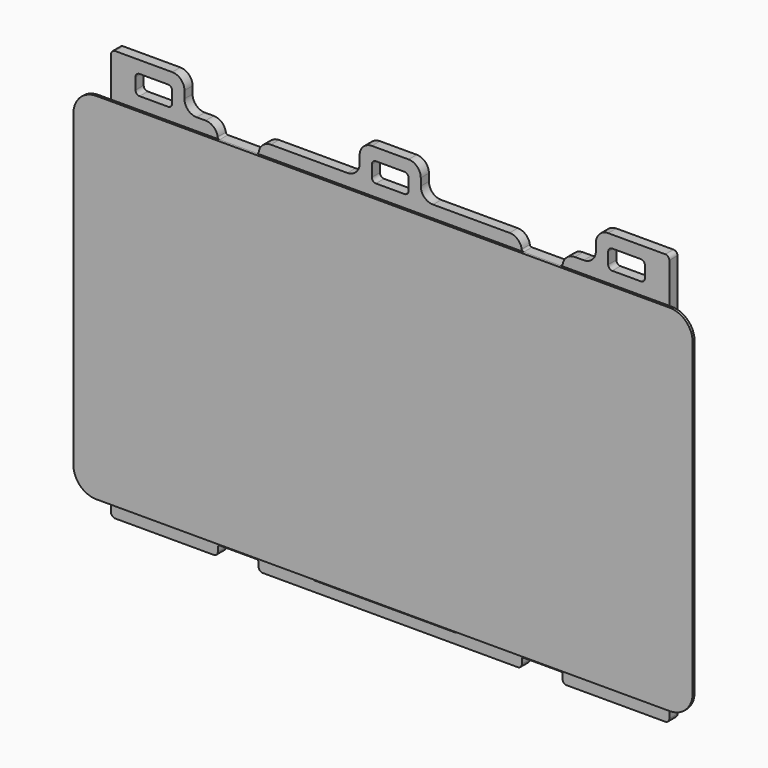
from build123d import *

# Parameters (mm, degrees)
F1_DEPTH   = 0.762
F2_W       = 166.2938
F2_H       = 100.7999
F3_DEPTH   = 5.08
F4_W       = 14.478
F4_H       = 7.874
F4_R       = 1.27
F4_W_2     = 7.874
F4_H_2     = 14.478
F5_DEPTH   = 2.413
F6_SIZE2   = 3.80999
F6_SIZE    = 2.41299
F6_2_SIZE2 = 3.80999
F6_2_SIZE  = 2.41299
F6_3_SIZE2 = 3.80999
F6_3_SIZE  = 2.41299
F6_4_SIZE2 = 3.80999
F6_4_SIZE  = 2.41299
F6_5_SIZE2 = 3.80999
F6_5_SIZE  = 2.41299
F6_6_SIZE2 = 3.80999
F6_6_SIZE  = 2.41299
F6_7_SIZE2 = 3.80999
F6_7_SIZE  = 2.41299
F6_8_SIZE2 = 3.80999
F6_8_SIZE  = 2.41299
F6_9_SIZE2 = 3.80999
F6_9_SIZE  = 2.41299
F7_SIZE2   = 3.80999
F7_SIZE    = 2.41299
F7_2_SIZE2 = 3.80999
F7_2_SIZE  = 2.41299
F7_3_SIZE2 = 3.80999
F7_3_SIZE  = 2.41299
F7_4_SIZE2 = 3.80999
F7_4_SIZE  = 2.41299
F7_5_SIZE2 = 3.80999
F7_5_SIZE  = 2.41299
F7_6_SIZE2 = 3.80999
F7_6_SIZE  = 2.41299
F7_7_SIZE2 = 3.80999
F7_7_SIZE  = 2.41299
F9_DEPTH   = 73.533
F11_DEPTH  = 64.2493
F12_W      = 40.005
F12_H      = 5.08
F13_DEPTH  = 3.2131
F15_DEPTH  = 3.175
F18_DEPTH  = 3.175
F19_R      = 0.635
F19_2_R    = 0.635


# Not quite as in the source:
# - a fillet or chamfer is up to 0.001 mm smaller than in the source, because OpenCascade refuses the exact size


with BuildPart() as f1:
    # F0 (on Front) → F1 (new body)
    with BuildSketch(Plane.XZ):
        with BuildLine():
            ThreePointArc((96.4565, 48.1965), (94.3734434278, 53.2254434278), (89.3445, 55.3085))
            Line((89.3445, 55.3085), (-89.3445, 55.3085))
            ThreePointArc((-89.3445, 55.3085), (-94.3734434278, 53.2254434278), (-96.4565, 48.1965))
            Line((-96.4565, 48.1965), (-96.4565, -48.1965))
            ThreePointArc((-96.4565, -48.1965), (-94.3734434278, -53.2254434278), (-89.3445, -55.3085))
            Line((-89.3445, -55.3085), (89.3445, -55.3085))
            ThreePointArc((89.3445, -55.3085), (94.3734434278, -53.2254434278), (96.4565, -48.1965))
            Line((96.4565, -48.1965), (96.4565, 48.1965))
        make_face()
    extrude(amount=F1_DEPTH)

    # F2 (on face) → F3 (join)
    with BuildSketch(Plane(origin=(0, 0, 0), x_dir=(-1, 0, 0), z_dir=(0, 1, 0))):
        with Locations((-1.6256, -1.69545)):
            Rectangle(F2_W, F2_H)
    extrude(amount=F3_DEPTH)

    # F4 (on face) → F5 (join)
    with BuildSketch(Plane(origin=(0, 5.08, 0), x_dir=(-1, 0, 0), z_dir=(0, 1, 0))):
        with Locations((-63.9699, 33.7185)):
            Rectangle(F4_W, F4_H)
        with Locations((-63.9699, 33.7185)):
            Circle(F4_R, mode=Mode.SUBTRACT)
        with Locations((-63.9699, -31.9405)):
            Rectangle(F4_W, F4_H)
        with Locations((-63.9699, -31.9405)):
            Circle(F4_R, mode=Mode.SUBTRACT)
        with Locations((62.2427, 33.7185)):
            Rectangle(F4_W, F4_H)
        with Locations((62.2427, 33.7185)):
            Circle(F4_R, mode=Mode.SUBTRACT)
        with Locations((62.2427, -31.9405)):
            Rectangle(F4_W, F4_H)
        with Locations((62.2427, -31.9405)):
            Circle(F4_R, mode=Mode.SUBTRACT)
        with Locations((-37.2872, 28.88996)):
            Rectangle(F4_W_2, F4_H_2)
        with Locations((-37.2872, 28.88996)):
            Circle(F4_R, mode=Mode.SUBTRACT)
        with Locations((19.0881, 28.88996)):
            Rectangle(F4_W_2, F4_H_2)
        with Locations((19.0881, 28.88996)):
            Circle(F4_R, mode=Mode.SUBTRACT)
        with Locations((-37.2872, -19.37004)):
            Rectangle(F4_W_2, F4_H_2)
        with Locations((-37.2872, -19.37004)):
            Circle(F4_R, mode=Mode.SUBTRACT)
        with Locations((19.0881, -19.37004)):
            Rectangle(F4_W_2, F4_H_2)
        with Locations((19.0881, -19.37004)):
            Circle(F4_R, mode=Mode.SUBTRACT)
    extrude(amount=F5_DEPTH)

    # F6 (size 2.413 and 3.81 in the source; OpenCascade refuses exactly that, so slightly less here)
    f6_edges = [f1.edges().sort_by_distance(p)[0] for p in [
        (56.7309, 7.493, 33.7185),
    ]]
    f6_side = f1.faces().sort_by_distance((56.7309, 6.2865, 33.7185))[0]
    chamfer(f6_edges, length=F6_SIZE, length2=F6_SIZE2, reference=f6_side)

    # F6#2 (size 2.413 and 3.81 in the source; OpenCascade refuses exactly that, so slightly less here)
    f6_2_edges = [f1.edges().sort_by_distance(p)[0] for p in [
        (71.2089, 7.493, 33.7185),
    ]]
    f6_2_side = f1.faces().sort_by_distance((71.2089, 6.2865, 33.7185))[0]
    chamfer(f6_2_edges, length=F6_2_SIZE, length2=F6_2_SIZE2, reference=f6_2_side)

    # F6#3 (size 2.413 and 3.81 in the source; OpenCascade refuses exactly that, so slightly less here)
    f6_3_edges = [f1.edges().sort_by_distance(p)[0] for p in [
        (56.7309, 7.493, -31.9405),
    ]]
    f6_3_side = f1.faces().sort_by_distance((56.7309, 6.2865, -31.9405))[0]
    chamfer(f6_3_edges, length=F6_3_SIZE, length2=F6_3_SIZE2, reference=f6_3_side)

    # F6#4 (size 2.413 and 3.81 in the source; OpenCascade refuses exactly that, so slightly less here)
    f6_4_edges = [f1.edges().sort_by_distance(p)[0] for p in [
        (37.2872, 7.493, -26.60904),
    ]]
    f6_4_side = f1.faces().sort_by_distance((37.2872, 6.2865, -26.60904))[0]
    chamfer(f6_4_edges, length=F6_4_SIZE, length2=F6_4_SIZE2, reference=f6_4_side)

    # F6#5 (size 2.413 and 3.81 in the source; OpenCascade refuses exactly that, so slightly less here)
    f6_5_edges = [f1.edges().sort_by_distance(p)[0] for p in [
        (37.2872, 7.493, 21.65096),
    ]]
    f6_5_side = f1.faces().sort_by_distance((37.2872, 6.2865, 21.65096))[0]
    chamfer(f6_5_edges, length=F6_5_SIZE, length2=F6_5_SIZE2, reference=f6_5_side)

    # F6#6 (size 2.413 and 3.81 in the source; OpenCascade refuses exactly that, so slightly less here)
    f6_6_edges = [f1.edges().sort_by_distance(p)[0] for p in [
        (-19.0881, 7.493, -26.60904),
    ]]
    f6_6_side = f1.faces().sort_by_distance((-19.0881, 6.2865, -26.60904))[0]
    chamfer(f6_6_edges, length=F6_6_SIZE, length2=F6_6_SIZE2, reference=f6_6_side)

    # F6#7 (size 2.413 and 3.81 in the source; OpenCascade refuses exactly that, so slightly less here)
    f6_7_edges = [f1.edges().sort_by_distance(p)[0] for p in [
        (-19.0881, 7.493, 21.65096),
    ]]
    f6_7_side = f1.faces().sort_by_distance((-19.0881, 6.2865, 21.65096))[0]
    chamfer(f6_7_edges, length=F6_7_SIZE, length2=F6_7_SIZE2, reference=f6_7_side)

    # F6#8 (size 2.413 and 3.81 in the source; OpenCascade refuses exactly that, so slightly less here)
    f6_8_edges = [f1.edges().sort_by_distance(p)[0] for p in [
        (-69.4817, 7.493, 33.7185),
    ]]
    f6_8_side = f1.faces().sort_by_distance((-69.4817, 6.2865, 33.7185))[0]
    chamfer(f6_8_edges, length=F6_8_SIZE, length2=F6_8_SIZE2, reference=f6_8_side)

    # F6#9 (size 2.413 and 3.81 in the source; OpenCascade refuses exactly that, so slightly less here)
    f6_9_edges = [f1.edges().sort_by_distance(p)[0] for p in [
        (-69.4817, 7.493, -31.9405),
    ]]
    f6_9_side = f1.faces().sort_by_distance((-69.4817, 6.2865, -31.9405))[0]
    chamfer(f6_9_edges, length=F6_9_SIZE, length2=F6_9_SIZE2, reference=f6_9_side)

    # F7 (size 2.413 and 3.81 in the source; OpenCascade refuses exactly that, so slightly less here)
    f7_edges = [f1.edges().sort_by_distance(p)[0] for p in [
        (37.2872, 7.493, 36.12896),
    ]]
    f7_side = f1.faces().sort_by_distance((37.2872, 6.2865, 36.12896))[0]
    chamfer(f7_edges, length=F7_SIZE, length2=F7_SIZE2, reference=f7_side)

    # F7#2 (size 2.413 and 3.81 in the source; OpenCascade refuses exactly that, so slightly less here)
    f7_2_edges = [f1.edges().sort_by_distance(p)[0] for p in [
        (71.2089, 7.493, -31.9405),
    ]]
    f7_2_side = f1.faces().sort_by_distance((71.2089, 6.2865, -31.9405))[0]
    chamfer(f7_2_edges, length=F7_2_SIZE, length2=F7_2_SIZE2, reference=f7_2_side)

    # F7#3 (size 2.413 and 3.81 in the source; OpenCascade refuses exactly that, so slightly less here)
    f7_3_edges = [f1.edges().sort_by_distance(p)[0] for p in [
        (37.2872, 7.493, -12.13104),
    ]]
    f7_3_side = f1.faces().sort_by_distance((37.2872, 6.2865, -12.13104))[0]
    chamfer(f7_3_edges, length=F7_3_SIZE, length2=F7_3_SIZE2, reference=f7_3_side)

    # F7#4 (size 2.413 and 3.81 in the source; OpenCascade refuses exactly that, so slightly less here)
    f7_4_edges = [f1.edges().sort_by_distance(p)[0] for p in [
        (-19.0881, 7.493, -12.13104),
    ]]
    f7_4_side = f1.faces().sort_by_distance((-19.0881, 6.2865, -12.13104))[0]
    chamfer(f7_4_edges, length=F7_4_SIZE, length2=F7_4_SIZE2, reference=f7_4_side)

    # F7#5 (size 2.413 and 3.81 in the source; OpenCascade refuses exactly that, so slightly less here)
    f7_5_edges = [f1.edges().sort_by_distance(p)[0] for p in [
        (-19.0881, 7.493, 36.12896),
    ]]
    f7_5_side = f1.faces().sort_by_distance((-19.0881, 6.2865, 36.12896))[0]
    chamfer(f7_5_edges, length=F7_5_SIZE, length2=F7_5_SIZE2, reference=f7_5_side)

    # F7#6 (size 2.413 and 3.81 in the source; OpenCascade refuses exactly that, so slightly less here)
    f7_6_edges = [f1.edges().sort_by_distance(p)[0] for p in [
        (-55.0037, 7.493, 33.7185),
    ]]
    f7_6_side = f1.faces().sort_by_distance((-55.0037, 6.2865, 33.7185))[0]
    chamfer(f7_6_edges, length=F7_6_SIZE, length2=F7_6_SIZE2, reference=f7_6_side)

    # F7#7 (size 2.413 and 3.81 in the source; OpenCascade refuses exactly that, so slightly less here)
    f7_7_edges = [f1.edges().sort_by_distance(p)[0] for p in [
        (-55.0037, 7.493, -31.9405),
    ]]
    f7_7_side = f1.faces().sort_by_distance((-55.0037, 6.2865, -31.9405))[0]
    chamfer(f7_7_edges, length=F7_7_SIZE, length2=F7_7_SIZE2, reference=f7_7_side)

    # F8 (on face) → F9 (cut, through all)
    with BuildSketch(Plane.XY.offset(37.6555)):
        Polygon((-65.5980324895, 7.239), (-69.0069798579, 5.08), (-55.4784201421, 5.08), (-58.8873675105, 7.239), align=None)
        Polygon((60.6145675105, 7.239), (57.2056201421, 5.08), (70.7341798579, 5.08), (67.3252324895, 7.239), align=None)
    extrude(amount=-F9_DEPTH, mode=Mode.SUBTRACT)

    # F10 (on face) → F11 (cut, through all)
    with BuildSketch(Plane(origin=(-23.0251, 0, 0), x_dir=(0, -1, 0), z_dir=(-1, 0, 0))):
        Polygon((-7.239, -22.7253724895), (-5.08, -26.1343198579), (-5.08, -12.6057601421), (-7.239, -16.0147075105), align=None)
        Polygon((-7.239, 25.5346275105), (-5.08, 22.1256801421), (-5.08, 35.6542398579), (-7.239, 32.2452924895), align=None)
    extrude(amount=-F11_DEPTH, mode=Mode.SUBTRACT)

    # F12 (on face) → F13 (join, through all)
    with BuildSketch(Plane(origin=(0, 0, -52.0954), x_dir=(1, 0, 0), z_dir=(0, 0, -1))):
        with Locations((-0.0508, -2.54)):
            Rectangle(F12_W, F12_H)
    extrude(amount=F13_DEPTH)


with BuildPart() as f15:
    # F14 (on face) → F15 (new body)
    with BuildSketch(Plane(origin=(0, 0, 0), x_dir=(-1, 0, 0), z_dir=(0, 1, 0))):
        with BuildLine():
            Line((-84.7725, 48.7045), (81.5213, 48.7045))
            Line((81.5213, 48.7045), (81.5213, 59.1185))
            Line((81.5213, 59.1185), (81.5213, 65.2145))
            ThreePointArc((81.5213, 65.2145), (80.4053768363, 67.9085768363), (77.7113, 69.0245))
            Line((77.7113, 69.0245), (66.2813, 69.0245))
            ThreePointArc((66.2813, 69.0245), (63.5872231637, 67.9085768363), (62.4713, 65.2145))
            Line((62.4713, 65.2145), (62.4713, 62.9285))
            ThreePointArc((62.4713, 62.9285), (61.3553768363, 60.2344231637), (58.6613, 59.1185))
            Line((58.6613, 59.1185), (55.88635, 59.1185))
            ThreePointArc((55.88635, 59.1185), (53.1922731637, 58.0025768363), (52.07635, 55.3085))
            Line((52.07635, 55.3085), (39.37635, 55.3085))
            ThreePointArc((39.37635, 55.3085), (38.2604268363, 58.0025768363), (35.56635, 59.1185))
            Line((35.56635, 59.1185), (11.7094, 59.1185))
            ThreePointArc((11.7094, 59.1185), (9.0153231637, 60.2344231637), (7.8994, 62.9285))
            Line((7.8994, 62.9285), (7.8994, 65.2145))
            ThreePointArc((7.8994, 65.2145), (6.7834768363, 67.9085768363), (4.0894, 69.0245))
            Line((4.0894, 69.0245), (-7.3406, 69.0245))
            ThreePointArc((-7.3406, 69.0245), (-10.0346768363, 67.9085768363), (-11.1506, 65.2145))
            Line((-11.1506, 65.2145), (-11.1506, 62.9285))
            ThreePointArc((-11.1506, 62.9285), (-12.2665231637, 60.2344231637), (-14.9606, 59.1185))
            Line((-14.9606, 59.1185), (-38.81755, 59.1185))
            ThreePointArc((-38.81755, 59.1185), (-41.5116268363, 58.0025768363), (-42.62755, 55.3085))
            Line((-42.62755, 55.3085), (-55.32755, 55.3085))
            ThreePointArc((-55.32755, 55.3085), (-56.4434731637, 58.0025768363), (-59.13755, 59.1185))
            Line((-59.13755, 59.1185), (-61.9125, 59.1185))
            ThreePointArc((-61.9125, 59.1185), (-64.6065768363, 60.2344231637), (-65.7225, 62.9285))
            Line((-65.7225, 62.9285), (-65.7225, 65.2145))
            ThreePointArc((-65.7225, 65.2145), (-66.8384231637, 67.9085768363), (-69.5325, 69.0245))
            Line((-69.5325, 69.0245), (-80.9625, 69.0245))
            ThreePointArc((-80.9625, 69.0245), (-83.6565768363, 67.9085768363), (-84.7725, 65.2145))
            Line((-84.7725, 65.2145), (-84.7725, 59.1185))
            Line((-84.7725, 59.1185), (-84.7725, 48.7045))
        make_face()
        with BuildLine():
            Line((-79.6925, 65.2145), (-70.8025, 65.2145))
            ThreePointArc((-70.8025, 65.2145), (-69.9044743879, 64.8425256121), (-69.5325, 63.9445))
            Line((-69.5325, 63.9445), (-69.5325, 60.3885))
            ThreePointArc((-69.5325, 60.3885), (-69.9044743879, 59.4904743879), (-70.8025, 59.1185))
            Line((-70.8025, 59.1185), (-79.6925, 59.1185))
            ThreePointArc((-79.6925, 59.1185), (-80.5905256121, 59.4904743879), (-80.9625, 60.3885))
            Line((-80.9625, 60.3885), (-80.9625, 63.9445))
            ThreePointArc((-80.9625, 63.9445), (-80.5905256121, 64.8425256121), (-79.6925, 65.2145))
        make_face(mode=Mode.SUBTRACT)
        with BuildLine():
            Line((-6.0706, 65.2145), (2.8194, 65.2145))
            ThreePointArc((2.8194, 65.2145), (3.7174256121, 64.8425256121), (4.0894, 63.9445))
            Line((4.0894, 63.9445), (4.0894, 60.3885))
            ThreePointArc((4.0894, 60.3885), (3.7174256121, 59.4904743879), (2.8194, 59.1185))
            Line((2.8194, 59.1185), (-6.0706, 59.1185))
            ThreePointArc((-6.0706, 59.1185), (-6.9686256121, 59.4904743879), (-7.3406, 60.3885))
            Line((-7.3406, 60.3885), (-7.3406, 63.9445))
            ThreePointArc((-7.3406, 63.9445), (-6.9686256121, 64.8425256121), (-6.0706, 65.2145))
        make_face(mode=Mode.SUBTRACT)
        with BuildLine():
            Line((67.5513, 65.2145), (76.4413, 65.2145))
            ThreePointArc((76.4413, 65.2145), (77.3393256121, 64.8425256121), (77.7113, 63.9445))
            Line((77.7113, 63.9445), (77.7113, 60.3885))
            ThreePointArc((77.7113, 60.3885), (77.3393256121, 59.4904743879), (76.4413, 59.1185))
            Line((76.4413, 59.1185), (67.5513, 59.1185))
            ThreePointArc((67.5513, 59.1185), (66.6532743879, 59.4904743879), (66.2813, 60.3885))
            Line((66.2813, 60.3885), (66.2813, 63.9445))
            ThreePointArc((66.2813, 63.9445), (66.6532743879, 64.8425256121), (67.5513, 65.2145))
        make_face(mode=Mode.SUBTRACT)
        with BuildLine():
            Line((81.5213, 59.1185), (81.5213, 48.7045))
            Line((81.5213, 48.7045), (82.1563, 48.7045))
            Line((82.1563, 48.7045), (82.1563, 46.7995))
            ThreePointArc((82.1563, 46.7995), (82.5282743879, 45.9014743879), (83.4263, 45.5295))
            Line((83.4263, 45.5295), (84.0613, 45.5295))
            ThreePointArc((84.0613, 45.5295), (84.9593256121, 45.9014743879), (85.3313, 46.7995))
            Line((85.3313, 46.7995), (85.3313, 67.7545))
            ThreePointArc((85.3313, 67.7545), (84.9593256121, 68.6525256121), (84.0613, 69.0245))
            Line((84.0613, 69.0245), (81.5213, 69.0245))
            Line((81.5213, 69.0245), (77.7113, 69.0245))
            ThreePointArc((77.7113, 69.0245), (80.4053768363, 67.9085768363), (81.5213, 65.2145))
            Line((81.5213, 65.2145), (81.5213, 59.1185))
        make_face()
        with BuildLine():
            Line((-85.4075, 48.7045), (-84.7725, 48.7045))
            Line((-84.7725, 48.7045), (-84.7725, 59.1185))
            Line((-84.7725, 59.1185), (-84.7725, 65.2145))
            Line((-84.7725, 65.2145), (-84.7725, 69.0245))
            Line((-84.7725, 69.0245), (-87.3125, 69.0245))
            ThreePointArc((-87.3125, 69.0245), (-88.2105256121, 68.6525256121), (-88.5825, 67.7545))
            Line((-88.5825, 67.7545), (-88.5825, 46.7995))
            ThreePointArc((-88.5825, 46.7995), (-88.2105256121, 45.9014743879), (-87.3125, 45.5295))
            Line((-87.3125, 45.5295), (-86.6775, 45.5295))
            ThreePointArc((-86.6775, 45.5295), (-85.7794743879, 45.9014743879), (-85.4075, 46.7995))
            Line((-85.4075, 46.7995), (-85.4075, 48.7045))
        make_face()
        with BuildLine():
            Line((-84.7725, 69.0245), (-84.7725, 65.2145))
            ThreePointArc((-84.7725, 65.2145), (-83.6565768363, 67.9085768363), (-80.9625, 69.0245))
            Line((-80.9625, 69.0245), (-84.7725, 69.0245))
        make_face()
    extrude(amount=F15_DEPTH)

    # F19#2
    f19_2_edges = [f15.edges().sort_by_distance(p)[0] for p in [
        (42.62755, 1.5875, 55.3085),
        (55.32755, 1.5875, 55.3085),
        (-39.37635, 1.5875, 55.3085),
        (-52.07635, 1.5875, 55.3085),
    ]]
    fillet(f19_2_edges, radius=F19_2_R)


with BuildPart() as f18:
    # F17 (on face) → F18 (new body)
    with BuildSketch(Plane(origin=(0, 0, 0), x_dir=(-1, 0, 0), z_dir=(0, 1, 0))):
        with BuildLine():
            ThreePointArc((-87.3125, -48.9204), (-88.2105256121, -49.2923743879), (-88.5825, -50.1904))
            Line((-88.5825, -50.1904), (-88.5825, -57.9012928972))
            ThreePointArc((-88.5825, -57.9012928972), (-88.2105256121, -58.7993185093), (-87.3125, -59.1712928972))
            Line((-87.3125, -59.1712928972), (-84.1375, -59.1712928972))
            Line((-84.1375, -59.1712928972), (-56.59755, -59.1712928972))
            ThreePointArc((-56.59755, -59.1712928972), (-55.6995243879, -58.7993185093), (-55.32755, -57.9012928972))
            Line((-55.32755, -57.9012928972), (-55.32755, -55.9962928972))
            Line((-55.32755, -55.9962928972), (-42.62755, -55.9962928972))
            Line((-42.62755, -55.9962928972), (-42.62755, -57.9012928972))
            ThreePointArc((-42.62755, -57.9012928972), (-42.2555756121, -58.7993185093), (-41.35755, -59.1712928972))
            Line((-41.35755, -59.1712928972), (38.10635, -59.1712928972))
            ThreePointArc((38.10635, -59.1712928972), (39.0043756121, -58.7993185093), (39.37635, -57.9012928972))
            Line((39.37635, -57.9012928972), (39.37635, -55.9962928972))
            Line((39.37635, -55.9962928972), (52.07635, -55.9962928972))
            Line((52.07635, -55.9962928972), (52.07635, -57.9012928972))
            ThreePointArc((52.07635, -57.9012928972), (52.4483243879, -58.7993185093), (53.34635, -59.1712928972))
            Line((53.34635, -59.1712928972), (84.0613, -59.1712928972))
            ThreePointArc((84.0613, -59.1712928972), (84.9593256121, -58.7993185093), (85.3313, -57.9012928972))
            Line((85.3313, -57.9012928972), (85.3313, -50.1904))
            ThreePointArc((85.3313, -50.1904), (84.9593256121, -49.2923743879), (84.0613, -48.9204))
            Line((84.0613, -48.9204), (83.4263, -48.9204))
            ThreePointArc((83.4263, -48.9204), (82.5282743879, -49.2923743879), (82.1563, -50.1904))
            Line((82.1563, -50.1904), (82.1563, -52.0954))
            Line((82.1563, -52.0954), (23.8633, -52.0954))
            ThreePointArc((23.8633, -52.0954), (22.9652743879, -52.4673743879), (22.5933, -53.3654))
            Line((22.5933, -53.3654), (22.5933, -55.9962928972))
            Line((22.5933, -55.9962928972), (-22.4917, -55.9962928972))
            Line((-22.4917, -55.9962928972), (-22.4917, -53.3654))
            ThreePointArc((-22.4917, -53.3654), (-22.8636743879, -52.4673743879), (-23.7617, -52.0954))
            Line((-23.7617, -52.0954), (-84.1375, -52.0954))
            Line((-84.1375, -52.0954), (-85.4075, -52.0954))
            Line((-85.4075, -52.0954), (-85.4075, -50.1904))
            ThreePointArc((-85.4075, -50.1904), (-85.7794743879, -49.2923743879), (-86.6775, -48.9204))
            Line((-86.6775, -48.9204), (-87.3125, -48.9204))
        make_face()
    extrude(amount=F18_DEPTH)

    # F19
    f19_edges = [f18.edges().sort_by_distance(p)[0] for p in [
        (22.4917, 1.5875, -55.996293),
        (-22.5933, 1.5875, -55.996293),
        (55.32755, 1.5875, -55.996293),
        (42.62755, 1.5875, -55.996293),
        (-52.07635, 1.5875, -55.996293),
        (-39.37635, 1.5875, -55.996293),
    ]]
    fillet(f19_edges, radius=F19_R)


solid = Compound([f1.part, f15.part, f18.part])
